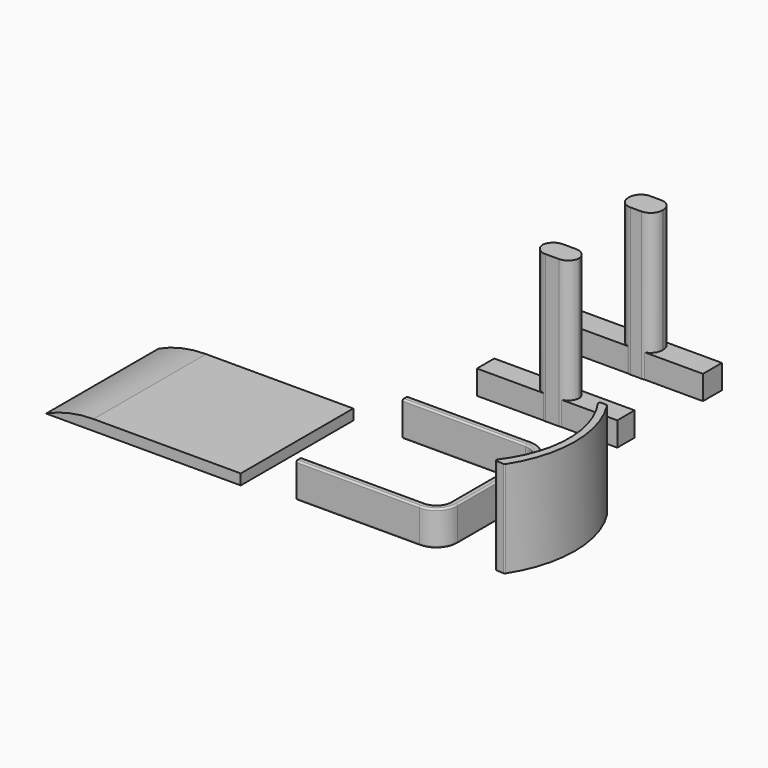
from build123d import *

# Parameters (mm, degrees)
F5_DEPTH       = 25.4
F6_W           = 51.3728456572
F6_H           = 37.123337388
F7_DEPTH       = 2.794
F8_T1_DEPTH    = 99.7075344175
F9_W           = 37.8610342741
F9_H           = 6.2647759914
F10_DEPTH      = 6.35
F9_W_2         = 37.0438918471
F9_H_2         = 5.7200118899
F11_W          = 8.9951548725
F11_H          = 6.4901784062
F12_DEPTH      = 38.862
F11_W_2        = 9.6783321351
F11_H_2        = 5.6931376457
F13_F1_R       = 3.0660512242
F13_F2_R       = 3.0660512242
F13_F3_R       = 3.0660512242
F13_F4_R       = 3.0660512242
F13_2_T1_DEPTH = 54.1922561211


# Not quite as in the source:
# - a fillet or chamfer that OpenCascade refuses, or shapes differently, is made with other operations: its cross-section is extruded or revolved along the edge and cut away or added


with BuildPart() as f2:
    # F2: sweep along a path in F0
    with BuildLine(Plane.XY) as f2_path:
        Line((0, 0), (32.4741261244, 0))
        ThreePointArc((32.4741261244, 0), (35.1682029607, -1.1159231637), (36.2841261244, -3.81))
        Line((36.2841261244, -3.81), (36.2841261244, -29.4484232092))
        ThreePointArc((36.2841261244, -29.4484232092), (35.1682029607, -32.1425000455), (32.4741261244, -33.2584232092))
        Line((32.4741261244, -33.2584232092), (0, -33.2584232092))
    # F1 (on Right) → F2 (sweep)
    with BuildSketch(Plane.YZ):
        with BuildLine():
            Line((0, 8.7253075845), (0, 0.43095164))
            ThreePointArc((0, 0.43095164), (0.126222813, 0.126222813), (0.43095164, 0))
            Line((0.43095164, 0), (1.3450375525, 0))
            ThreePointArc((1.3450375525, 0), (1.6497663795, 0.126222813), (1.7759891925, 0.43095164))
            Line((1.7759891925, 0.43095164), (1.7759891925, 8.7253075845))
            ThreePointArc((1.7759891925, 8.7253075845), (1.6497663795, 9.0300364115), (1.3450375525, 9.1562592245))
            Line((1.3450375525, 9.1562592245), (0.43095164, 9.1562592245))
            ThreePointArc((0.43095164, 9.1562592245), (0.126222813, 9.0300364115), (0, 8.7253075845))
        make_face()
    sweep(path=f2_path.line)


with BuildPart() as f5:
    # F3 (on Top) → F5 (new body)
    with BuildSketch(Plane.XY):
        with BuildLine():
            ThreePointArc((53.7307702021, -33.8673758858), (53.9602055935, -33.8170389493), (54.1338617807, -33.658868362))
            ThreePointArc((54.1338617807, -33.658868362), (59.0379747248, -16.932750892), (54.1264548633, -0.2088069181))
            ThreePointArc((54.1264548633, -0.2088069181), (53.9619320492, -0.0556032477), (53.7441078084, 0))
            Line((53.7441078084, 0), (52.4662340509, 0))
            ThreePointArc((52.4662340509, 0), (52.0623861341, -0.2460332441), (52.0958026022, -0.7177416675))
            ThreePointArc((52.0958026022, -0.7177416675), (57.1389747881, -16.9727260502), (51.5711781882, -33.0555660979))
            ThreePointArc((51.5711781882, -33.0555660979), (51.5212198267, -33.5232749621), (51.9122386741, -33.7847165054))
            Line((51.9122386741, -33.7847165054), (53.7307702021, -33.8673758858))
        make_face()
    extrude(amount=F5_DEPTH)


with BuildPart() as f7:
    # F6 (on Top) → F7 (new body)
    with BuildSketch(Plane.XY):
        with Locations((-38.7038192712, -18.561668694)):
            Rectangle(F6_W, F6_H)
    extrude(amount=F7_DEPTH)

    # F8: fillet of radius 29.4340917525 on 1 edges, made by hand

    # F8_s2 → F8_t1 (cut)
    with BuildSketch(Plane.XZ.offset(-31.2920985147)):
        with BuildLine():
            ThreePointArc((-64.3902420998, 0), (-58.2858457679, 2.0870092345), (-51.8734026939, 2.794))
            Line((-51.8734026939, 2.794), (-64.3902420998, 2.794))
            Line((-64.3902420998, 2.794), (-64.3902420998, 0))
        make_face()
    extrude(amount=F8_T1_DEPTH, mode=Mode.SUBTRACT)


with BuildPart() as f10:
    # F9 (on Top) → F10 (new body)
    with BuildSketch(Plane.XY):
        with Locations((18.9305171371, 54.8848770559)):
            Rectangle(F9_W, F9_H)
    extrude(amount=F10_DEPTH)


with BuildPart() as f10b:
    # F9 (on Top) → F10, piece 2 (new body)
    with BuildSketch(Plane.XY):
        with Locations((18.5219459236, 27.3743439466)):
            Rectangle(F9_W_2, F9_H_2)
    extrude(amount=F10_DEPTH)


with BuildPart() as f12:
    # F11 (on Top) → F12 (new body)
    with BuildSketch(Plane.XY):
        with Locations((20.2516885474, 54.9109317362)):
            Rectangle(F11_W, F11_H)
    extrude(amount=F12_DEPTH)

    # F13: fillet of radius 3.0660512242 on 4 edges, made by hand

    # F13_f1
    f13_f1_edges = [f12.edges().sort_by_distance(p)[0] for p in [
        (24.7492659837, 58.1560209394, 19.431),
    ]]
    fillet(f13_f1_edges, radius=F13_F1_R)

    # F13_f2
    f13_f2_edges = [f12.edges().sort_by_distance(p)[0] for p in [
        (15.7541111112, 58.1560209394, 19.431),
    ]]
    fillet(f13_f2_edges, radius=F13_F2_R)

    # F13_f3
    f13_f3_edges = [f12.edges().sort_by_distance(p)[0] for p in [
        (15.7541111112, 51.6658425331, 19.431),
    ]]
    fillet(f13_f3_edges, radius=F13_F3_R)

    # F13_f4
    f13_f4_edges = [f12.edges().sort_by_distance(p)[0] for p in [
        (24.7492659837, 51.6658425331, 19.431),
    ]]
    fillet(f13_f4_edges, radius=F13_F4_R)


with BuildPart() as f12b:
    # F11 (on Top) → F12, piece 2 (new body)
    with BuildSketch(Plane.XY):
        with Locations((19.9100999162, 27.2992197424)):
            Rectangle(F11_W_2, F11_H_2)
    extrude(amount=F12_DEPTH)

    # F13#2: fillet of radius 3.0660512242 on 4 edges, made by hand

    # F13_2_s2 → F13_2_t1 (cut)
    with BuildSketch(Plane.XY.offset(-7.6651280605)):
        with BuildLine():
            ThreePointArc((15.0709338486, 27.5187021438), (15.9689594607, 25.3506765317), (18.1369850728, 24.4526509196))
            Line((18.1369850728, 24.4526509196), (15.0709338486, 24.4526509196))
            Line((15.0709338486, 24.4526509196), (15.0709338486, 27.5187021438))
        make_face()
        with BuildLine():
            ThreePointArc((21.6832147595, 24.4526509196), (23.8512403716, 25.3506765317), (24.7492659837, 27.5187021438))
            Line((24.7492659837, 27.5187021438), (24.7492659837, 24.4526509196))
            Line((24.7492659837, 24.4526509196), (21.6832147595, 24.4526509196))
        make_face()
        with BuildLine():
            ThreePointArc((21.6832147595, 30.1457885653), (23.8512403716, 29.2477629532), (24.7492659837, 27.0797373411))
            Line((24.7492659837, 27.0797373411), (24.7492659837, 30.1457885653))
            Line((24.7492659837, 30.1457885653), (21.6832147595, 30.1457885653))
        make_face()
        with BuildLine():
            ThreePointArc((18.1369850728, 30.1457885653), (15.9689594607, 29.2477629532), (15.0709338486, 27.0797373411))
            Line((15.0709338486, 27.0797373411), (15.0709338486, 30.1457885653))
            Line((15.0709338486, 30.1457885653), (18.1369850728, 30.1457885653))
        make_face()
    extrude(amount=F13_2_T1_DEPTH, mode=Mode.SUBTRACT)


solid = Compound([f2.part, f5.part, f7.part, f10.part, f10b.part, f12.part, f12b.part])
